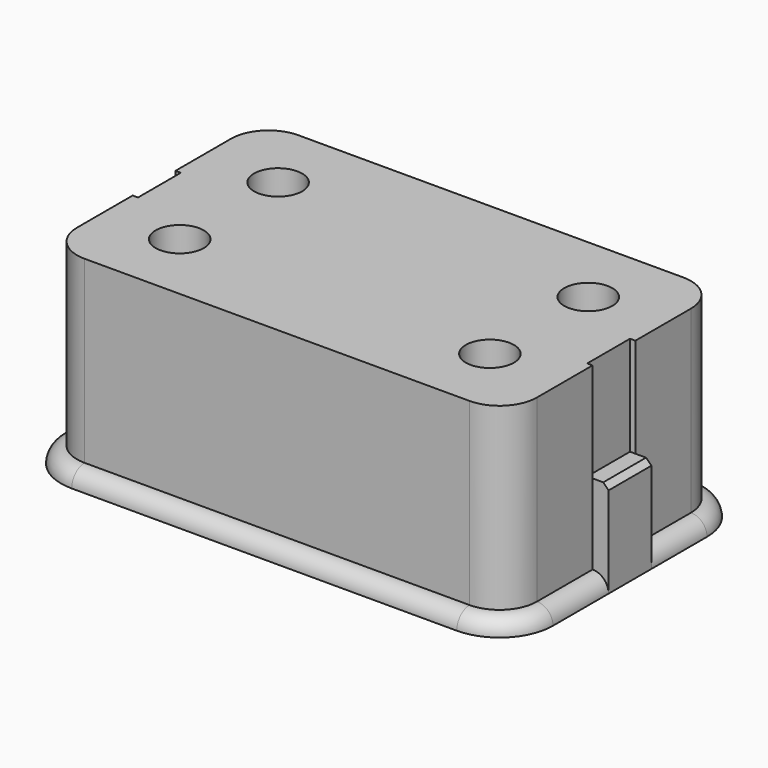
from build123d import *

# Parameters (mm, degrees)
F2_DEPTH  = 3
F1_R      = 2.5
F1_R_2    = 1.25
F3_DEPTH  = 10
F4_SIZE2  = 3
F4_SIZE   = 2
F5_R      = 2.99999
F7_W      = 10
F7_H      = 18
F8_DEPTH  = 4
F10_SIZE  = 1
F11_DEPTH = 33.6


# Not quite as in the source:
# - a fillet or chamfer is up to 0.001 mm smaller than in the source, because OpenCascade refuses the exact size


with BuildPart() as f2:
    # F0 (on Top) → F2 (new body)
    with BuildSketch(Plane.XY):
        with BuildLine():
            ThreePointArc((46, 18), (43.0710678119, 25.0710678119), (36, 28))
            Line((36, 28), (-36, 28))
            ThreePointArc((-36, 28), (-43.0710678119, 25.0710678119), (-46, 18))
            Line((-46, 18), (-46, -18))
            ThreePointArc((-46, -18), (-43.0710678119, -25.0710678119), (-36, -28))
            Line((-36, -28), (36, -28))
            ThreePointArc((36, -28), (43.0710678119, -25.0710678119), (46, -18))
            Line((46, -18), (46, 18))
        make_face()
    extrude(amount=F2_DEPTH)

    # F1 (on Top) → F3 (join)
    with BuildSketch(Plane.XY):
        with Locations((-29, 11.5)):
            Circle(F1_R)
        with Locations((-29, 11.5)):
            Circle(F1_R_2, mode=Mode.SUBTRACT)
        with Locations((29, 11.5)):
            Circle(F1_R)
        with Locations((29, 11.5)):
            Circle(F1_R_2, mode=Mode.SUBTRACT)
        with Locations((-29, -11.5)):
            Circle(F1_R)
        with Locations((-29, -11.5)):
            Circle(F1_R_2, mode=Mode.SUBTRACT)
        with Locations((29, -11.5)):
            Circle(F1_R)
        with Locations((29, -11.5)):
            Circle(F1_R_2, mode=Mode.SUBTRACT)
    extrude(amount=F3_DEPTH)

    # F4
    f4_edges = [f2.edges().sort_by_distance(p)[0] for p in [
        (-31.5, 11.5, 3),
        (26.5, 11.5, 3),
        (26.5, -11.5, 3),
        (-31.5, -11.5, 3),
    ]]
    chamfer(f4_edges, length=F4_SIZE, length2=F4_SIZE2)

    # F5 (radius 3 in the source; OpenCascade refuses exactly that, so slightly less here)
    f5_edges = [f2.edges().sort_by_distance(p)[0] for p in [
        (0, 28, 3),
    ]]
    fillet(f5_edges, radius=F5_R)

    # F7 (on offset) → F8 (join)
    with BuildSketch(Plane.YZ.offset(46)):
        with Locations((0, 9)):
            Rectangle(F7_W, F7_H)
    extrude(amount=-F8_DEPTH)

    # F9: F2 across plane


with BuildPart() as f2_1:
    add(f2.part)
    add(f2.part.mirror(Plane.YZ))

    # F10
    f10_edges = [f2_1.edges().sort_by_distance(p)[0] for p in [
        (-46, 0, 18),
        (46, 0, 18),
    ]]
    chamfer(f10_edges, length=F10_SIZE)

    # F11 (add): a face of the model
    f11_faces = [f2_1.faces().sort_by_distance(p)[0] for p in [
        (0, 0, 3),
    ]]
    extrude(f11_faces, amount=F11_DEPTH)


solid = f2_1.part
